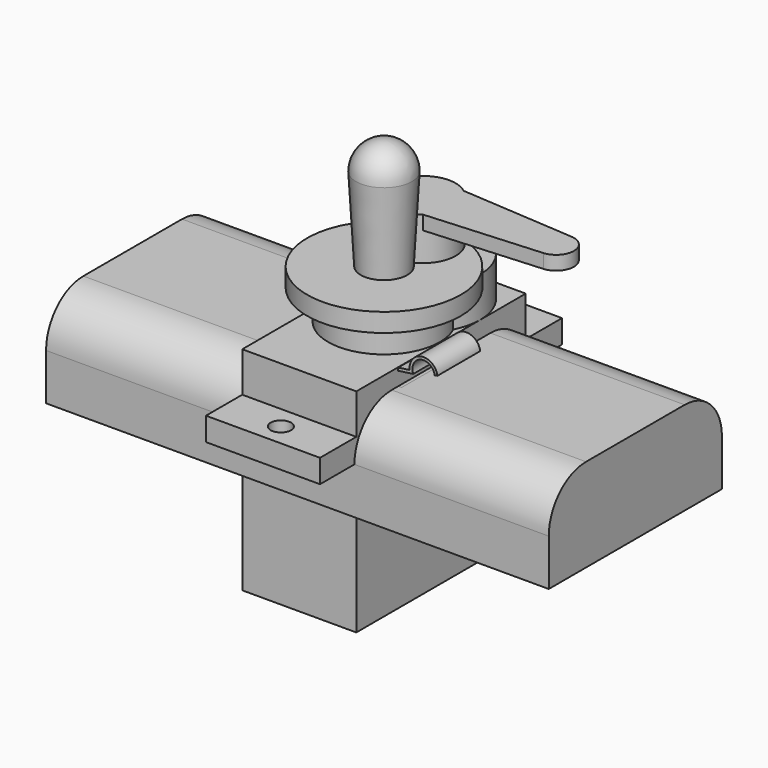
from build123d import *

# Parameters (mm, degrees)
F1_DEPTH  = 27
F4_W      = 11.5
F4_H      = 13
F5_DEPTH  = 13
F6_R      = 8.2561088494
F7_DEPTH  = 2
F8_W      = 12.25
F8_H      = 22.75
F9_DEPTH  = 16
F10_W     = 12.25
F10_H     = 32.5
F10_R     = 1.1
F11_DEPTH = 2.5
F12_W     = 12.25
F12_H     = 22.75
F13_DEPTH = 4.3
F15_DEPTH = 4.3
F16_R     = 3.5
F17_DEPTH = 5.5
F19_DEPTH = 1.5
F20_R     = 1
F21_DEPTH = 5.75


with BuildPart() as f1:
    # F0 (on Right) → F1 (new body, symmetric)
    with BuildSketch(Plane.YZ):
        with BuildLine():
            ThreePointArc((11.625, 0), (10.1605339059, 3.5355339059), (6.625, 5))
            Line((6.625, 5), (-6.625, 5))
            ThreePointArc((-6.625, 5), (-10.1605339059, 3.5355339059), (-11.625, 0))
            Line((-11.625, 0), (-11.625, -5))
            Line((-11.625, -5), (11.625, -5))
            Line((11.625, -5), (11.625, 0))
        make_face()
    extrude(amount=F1_DEPTH, both=True)


with BuildPart() as f3:
    # F2 (on Front) → F3 (revolve)
    with BuildSketch(Plane.XZ):
        with BuildLine():
            Line((0, 24), (0, 0))
            Line((0, 0), (6, 0))
            Line((6, 0), (6, 12))
            Line((6, 12), (2.5, 12))
            Line((2.5, 12), (3, 21))
            ThreePointArc((3, 21), (2.1213203436, 23.1213203436), (0, 24))
        make_face()
    revolve(axis=Axis((0, 0, 12), (0, 0, 1)))

    # F4 (on face) → F5 (join)
    with BuildSketch(Plane(origin=(0, 0, 0), x_dir=(1, 0, 0), z_dir=(0, 0, -1))):
        Rectangle(F4_W, F4_H)
    extrude(amount=F5_DEPTH)

    # F6 (on face) → F7 (join)
    with BuildSketch(Plane.XY.offset(12)):
        Circle(F6_R)
    extrude(amount=-F7_DEPTH)


with BuildPart() as f9:
    # F8 (on Top) → F9 (new body)
    with BuildSketch(Plane.XY):
        Rectangle(F8_W, F8_H)
    extrude(amount=-F9_DEPTH)

    # F10 (on face) → F11 (join)
    with BuildSketch(Plane.XY):
        Rectangle(F10_W, F10_H)
        with Locations((0, -13.85)):
            Circle(F10_R, mode=Mode.SUBTRACT)
        with Locations((0, 13.85)):
            Circle(F10_R, mode=Mode.SUBTRACT)
    extrude(amount=F11_DEPTH)

    # F12 (on face) → F13 (join)
    with BuildSketch(Plane.XY.offset(2.5)):
        Rectangle(F12_W, F12_H)
    extrude(amount=F13_DEPTH)

    # F14 (on face) → F15 (join)
    with BuildSketch(Plane.XY.offset(6.8)):
        with BuildLine():
            ThreePointArc((-2.7389294479, -0.2284934498), (0, -3.225), (2.7389294479, -0.2284934498))
            ThreePointArc((2.7389294479, -0.2284934498), (0, 11.375), (-2.7389294479, -0.2284934498))
        make_face()
    extrude(amount=F15_DEPTH)


with BuildPart() as f17:
    # F16 (on face) → F17 (new body)
    with BuildSketch(Plane.XY.offset(11.1)):
        with Locations((0, 5.25)):
            Circle(F16_R)
    extrude(amount=F17_DEPTH)

    # F18 (on face) → F19 (join)
    with BuildSketch(Plane.XY.offset(16.6)):
        with BuildLine():
            ThreePointArc((14.4271473678, 3.35), (16.2, 5.25), (14.4271473678, 7.15))
            Line((14.4271473678, 7.15), (2.1650635095, 8))
            Line((2.1650635095, 8), (2.1650635095, 2.5))
            Line((2.1650635095, 2.5), (14.4271473678, 3.35))
        make_face()
    extrude(amount=-F19_DEPTH)


with BuildPart() as f21:
    # F20 (on Front) → F21 (new body)
    with BuildSketch(Plane.XZ):
        Polygon((6.5, -5), (6.5, 5), (-4.3333333333, 5), (-6.5, 5), (-6.5, -5), align=None)
        with Locations((-3.375, 0)):
            Circle(F20_R, mode=Mode.SUBTRACT)
        with BuildLine():
            ThreePointArc((2.625, -1), (2.125, 0), (2.625, 1))
            Line((2.625, 1), (4.125, 1))
            ThreePointArc((4.125, 1), (4.625, 0), (4.125, -1))
            Line((4.125, -1), (2.625, -1))
        make_face(mode=Mode.SUBTRACT)
        with BuildLine():
            Line((-6.5, 5), (-4.3333333333, 5))
            Line((-4.3333333333, 5), (7.7415361299, 6.6881657329))
            ThreePointArc((7.7415361299, 6.6881657329), (8.5361228167, 8.3041868836), (10.0391424547, 7.3123076923))
            Line((10.0391424547, 7.3123076923), (10.3362527982, 7.3538461538))
            ThreePointArc((10.3362527982, 7.3538461538), (8.643008773, 8.6317055636), (7.3651493632, 6.9384615385))
            Line((7.3651493632, 6.9384615385), (-6.5, 5))
        make_face()
    extrude(amount=F21_DEPTH)


solid = Compound([f1.part, f3.part, f9.part, f17.part, f21.part])
